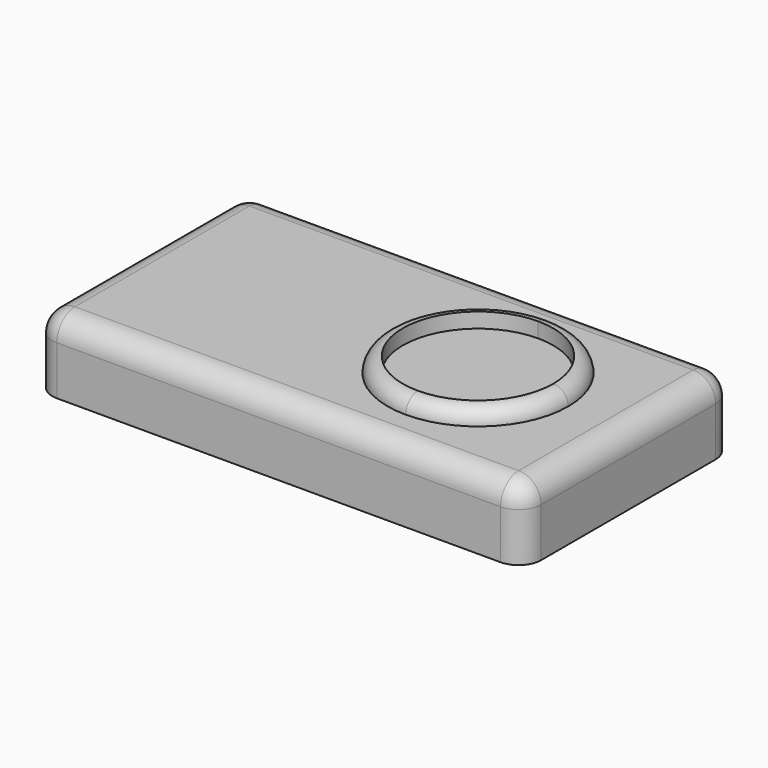
from build123d import *

# Parameters (mm, degrees)
F1_DEPTH = 9.5
F2_DEPTH = 11.5
F3_R     = 1.99999
F4_R     = 3


# Not quite as in the source:
# - a fillet or chamfer is up to 0.001 mm smaller than in the source, because OpenCascade refuses the exact size


with BuildPart() as f1:
    # F0 (on Top) → F1 (new body)
    with BuildSketch(Plane.XY):
        with BuildLine():
            Line((6.7996287718, 5.2781800885), (-38.2003712282, 5.2781800885))
            Line((-38.2003712282, 5.2781800885), (-38.2003712282, -29.7218199115))
            Line((-38.2003712282, -29.7218199115), (6.7996287718, -29.7218199115))
            Line((6.7996287718, -29.7218199115), (6.7996287718, -24.2218199115))
            ThreePointArc((6.7996287718, -24.2218199115), (-5.2003712282, -12.2218199115), (6.7996287718, -0.2218199115))
            Line((6.7996287718, -0.2218199115), (6.7996287718, 5.2781800885))
        make_face()
        with BuildLine():
            Line((26.7996287718, 5.2781800885), (6.7996287718, 5.2781800885))
            Line((6.7996287718, 5.2781800885), (6.7996287718, -0.2218199115))
            ThreePointArc((6.7996287718, -0.2218199115), (15.2849101461, -3.7365385373), (18.7996287718, -12.2218199115))
            Line((18.7996287718, -12.2218199115), (26.7996287718, -12.2218199115))
            Line((26.7996287718, -12.2218199115), (26.7996287718, 5.2781800885))
        make_face()
        with BuildLine():
            Line((6.7996287718, -24.2218199115), (6.7996287718, -29.7218199115))
            Line((6.7996287718, -29.7218199115), (26.7996287718, -29.7218199115))
            Line((26.7996287718, -29.7218199115), (26.7996287718, -12.2218199115))
            Line((26.7996287718, -12.2218199115), (18.7996287718, -12.2218199115))
            ThreePointArc((18.7996287718, -12.2218199115), (15.2849101461, -20.7071012858), (6.7996287718, -24.2218199115))
        make_face()
        with BuildLine():
            ThreePointArc((6.7996287718, -24.2218199115), (15.2849101461, -20.7071012858), (18.7996287718, -12.2218199115))
            Line((18.7996287718, -12.2218199115), (16.7996287718, -12.2218199115))
            ThreePointArc((16.7996287718, -12.2218199115), (13.8706965837, -19.2928877234), (6.7996287718, -22.2218199115))
            Line((6.7996287718, -22.2218199115), (6.7996287718, -24.2218199115))
        make_face()
        with BuildLine():
            ThreePointArc((18.7996287718, -12.2218199115), (15.2849101461, -3.7365385373), (6.7996287718, -0.2218199115))
            Line((6.7996287718, -0.2218199115), (6.7996287718, -2.2218199115))
            ThreePointArc((6.7996287718, -2.2218199115), (13.8706965837, -5.1507520997), (16.7996287718, -12.2218199115))
            Line((16.7996287718, -12.2218199115), (18.7996287718, -12.2218199115))
        make_face()
        with BuildLine():
            Line((6.7996287718, -2.2218199115), (6.7996287718, -0.2218199115))
            ThreePointArc((6.7996287718, -0.2218199115), (-5.2003712282, -12.2218199115), (6.7996287718, -24.2218199115))
            Line((6.7996287718, -24.2218199115), (6.7996287718, -22.2218199115))
            ThreePointArc((6.7996287718, -22.2218199115), (-3.2003712282, -12.2218199115), (6.7996287718, -2.2218199115))
        make_face()
        with BuildLine():
            Line((6.7996287718, -22.2218199115), (6.7996287718, -2.2218199115))
            ThreePointArc((6.7996287718, -2.2218199115), (-3.2003712282, -12.2218199115), (6.7996287718, -22.2218199115))
        make_face()
        with BuildLine():
            ThreePointArc((16.7996287718, -12.2218199115), (13.8706965837, -5.1507520997), (6.7996287718, -2.2218199115))
            Line((6.7996287718, -2.2218199115), (6.7996287718, -22.2218199115))
            ThreePointArc((6.7996287718, -22.2218199115), (13.8706965837, -19.2928877234), (16.7996287718, -12.2218199115))
        make_face()
    extrude(amount=F1_DEPTH)

    # F0 (on Top) → F2 (join)
    with BuildSketch(Plane.XY):
        with BuildLine():
            ThreePointArc((6.7996287718, -24.2218199115), (15.2849101461, -20.7071012858), (18.7996287718, -12.2218199115))
            Line((18.7996287718, -12.2218199115), (16.7996287718, -12.2218199115))
            ThreePointArc((16.7996287718, -12.2218199115), (13.8706965837, -19.2928877234), (6.7996287718, -22.2218199115))
            Line((6.7996287718, -22.2218199115), (6.7996287718, -24.2218199115))
        make_face()
        with BuildLine():
            ThreePointArc((18.7996287718, -12.2218199115), (15.2849101461, -3.7365385373), (6.7996287718, -0.2218199115))
            Line((6.7996287718, -0.2218199115), (6.7996287718, -2.2218199115))
            ThreePointArc((6.7996287718, -2.2218199115), (13.8706965837, -5.1507520997), (16.7996287718, -12.2218199115))
            Line((16.7996287718, -12.2218199115), (18.7996287718, -12.2218199115))
        make_face()
        with BuildLine():
            Line((6.7996287718, -2.2218199115), (6.7996287718, -0.2218199115))
            ThreePointArc((6.7996287718, -0.2218199115), (-5.2003712282, -12.2218199115), (6.7996287718, -24.2218199115))
            Line((6.7996287718, -24.2218199115), (6.7996287718, -22.2218199115))
            ThreePointArc((6.7996287718, -22.2218199115), (-3.2003712282, -12.2218199115), (6.7996287718, -2.2218199115))
        make_face()
    extrude(amount=F2_DEPTH)

    # F3 (radius 2 in the source; OpenCascade refuses exactly that, so slightly less here)
    f3_edges = [f1.edges().sort_by_distance(p)[0] for p in [
        (6.799629, -24.22182, 11.5),
    ]]
    fillet(f3_edges, radius=F3_R)

    # F4
    f4_edges = [f1.edges().sort_by_distance(p)[0] for p in [
        (-5.700371, -29.72182, 9.5),
        (26.799629, -12.22182, 9.5),
        (26.799629, -29.72182, 4.75),
        (-38.200371, -29.72182, 4.75),
        (-38.200371, -12.22182, 9.5),
        (-38.200371, 5.27818, 4.75),
        (26.799629, 5.27818, 4.75),
        (-5.700371, 5.27818, 9.5),
    ]]
    fillet(f4_edges, radius=F4_R)


solid = f1.part
